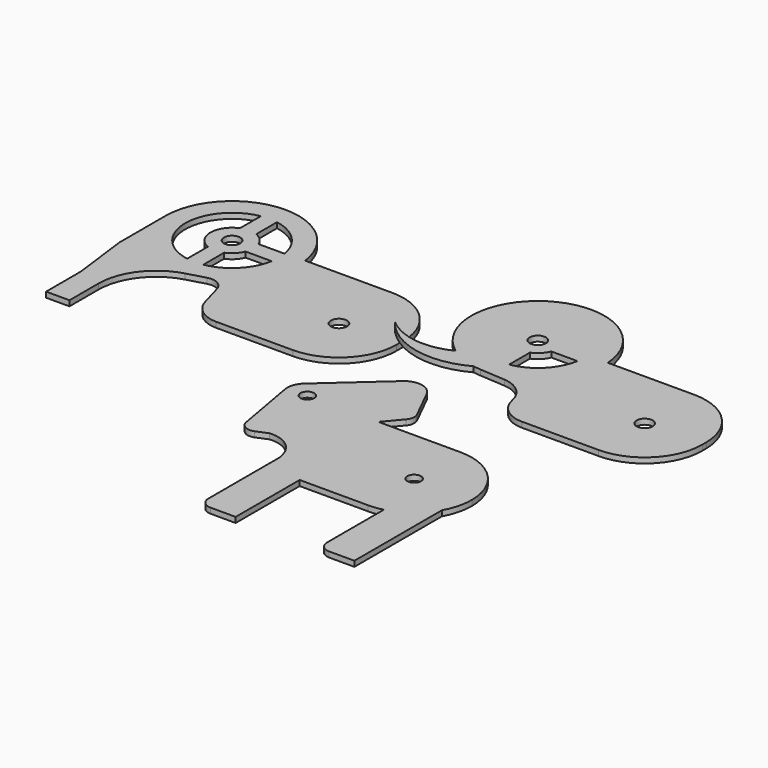
from build123d import *

# Parameters (mm, degrees)
F1_R     = 2.25
F2_DEPTH = 1.5
F3_R     = 2.25
F4_DEPTH = 1.5
F5_R     = 1.905
F6_DEPTH = 1.5


# Not quite as in the source:
# - a feature names something its author has since deleted; it is built from what else it names


with BuildPart() as f2:
    # F1 (on Top) → F2 (new body)
    with BuildSketch(Plane.XY):
        with BuildLine():
            Line((23.8478663564, 16.2219721824), (-0.3218308638, 16.2219721824))
            ThreePointArc((-0.3218308638, 16.2219721824), (-19.9050100488, 32.1794991216), (-37.1521336436, 13.7219721824))
            Line((-37.1521336436, 13.7219721824), (-37.1521336436, -2.2780278176))
            Line((-37.1521336436, -2.2780278176), (-35.1421336436, -18.2780278176))
            Line((-35.1421336436, -18.2780278176), (-35.1421336436, -30.2780278176))
            Line((-35.1421336436, -30.2780278176), (-28.6421336436, -30.2780278176))
            Line((-28.6421336436, -30.2780278176), (-28.6421336436, -20.1922246362))
            ThreePointArc((-28.6421336436, -20.1922246362), (-25.3982996099, -10.5340555633), (-16.9821049136, -4.7920736832))
            Line((-16.9821049136, -4.7920736832), (-11.9111882435, -3.3630206351))
            ThreePointArc((-11.9111882435, -3.3630206351), (-8.8710134123, -3.723464802), (-6.9761576878, -6.1280655559))
            Line((-6.9761576878, -6.1280655559), (-5.1951107108, -12.4480134526))
            ThreePointArc((-5.1951107108, -12.4480134526), (-2.3241197708, -16.6561108008), (2.5049647657, -18.2780278176))
            Line((2.5049647657, -18.2780278176), (23.8478663564, -18.2780278176))
            ThreePointArc((23.8478663564, -18.2780278176), (35.1615748554, -13.5917363166), (39.8478663564, -2.2780278176))
            Line((39.8478663564, -2.2780278176), (39.8478663564, 0.2219721824))
            ThreePointArc((39.8478663564, 0.2219721824), (35.1615748554, 11.5356806814), (23.8478663564, 16.2219721824))
        make_face()
        with Locations((23.8478663564, -2.2780278176)):
            Circle(F1_R, mode=Mode.SUBTRACT)
        with BuildLine():
            Line((-20.9021336436, 26.5257802097), (-20.9021336436, 19.2841210477))
            ThreePointArc((-20.9021336436, 19.2841210477), (-24.6521336436, 13.7219721824), (-20.9021336436, 8.1598233171))
            Line((-20.9021336436, 8.1598233171), (-20.9021336436, 0.9181641551))
            ThreePointArc((-20.9021336436, 0.9181641551), (-31.6521336436, 13.7219721824), (-20.9021336436, 26.5257802097))
        make_face(mode=Mode.SUBTRACT)
        with Locations((-18.6521336436, 13.7219721824)):
            Circle(F1_R, mode=Mode.SUBTRACT)
        with BuildLine():
            ThreePointArc((-16.4021336436, 8.1598233171), (-14.4094929565, 9.4793314953), (-13.0899847783, 11.4719721824))
            Line((-13.0899847783, 11.4719721824), (-5.8483256163, 11.4719721824))
            ThreePointArc((-5.8483256163, 11.4719721824), (-9.4597454882, 4.529584027), (-16.4021336436, 0.9181641551))
            Line((-16.4021336436, 0.9181641551), (-16.4021336436, 8.1598233171))
        make_face(mode=Mode.SUBTRACT)
        with BuildLine():
            ThreePointArc((-13.0899847783, 15.9719721824), (-14.4094929565, 17.9646128695), (-16.4021336436, 19.2841210477))
            Line((-16.4021336436, 19.2841210477), (-16.4021336436, 26.5257802097))
            ThreePointArc((-16.4021336436, 26.5257802097), (-9.4597454882, 22.9143603378), (-5.8483256163, 15.9719721824))
            Line((-5.8483256163, 15.9719721824), (-13.0899847783, 15.9719721824))
        make_face(mode=Mode.SUBTRACT)
    extrude(amount=F2_DEPTH)


with BuildPart() as f4:
    # F3 (on offset) → F4 (new body)
    with BuildSketch(Plane.XY.offset(3.5)):
        with BuildLine():
            Line((109.2000847661, 14.5111365989), (85.1578067274, 14.5111365989))
            ThreePointArc((85.1578067274, 14.5111365989), (85.1895122354, 13.8864939832), (85.2000847661, 13.2611365989))
            ThreePointArc((85.2000847661, 13.2611365989), (79.3391563377, -0.2482627146), (65.4699366786, -5.1979190563))
            Line((65.4699366786, -5.1979190563), (72.5876051284, -5.6722546017))
            ThreePointArc((72.5876051284, -5.6722546017), (77.0942321722, -7.4406386068), (79.7557246751, -11.4845633041))
            Line((79.7557246751, -11.4845633041), (80.1571076989, -12.9088490361))
            ThreePointArc((80.1571076989, -12.9088490361), (83.028098639, -17.1169463843), (87.8571831754, -18.7388634011))
            Line((87.8571831754, -18.7388634011), (109.2000847661, -18.7388634011))
            ThreePointArc((109.2000847661, -18.7388634011), (120.5137932651, -14.0525719001), (125.2000847661, -2.7388634011))
            Line((125.2000847661, -2.7388634011), (125.2000847661, -1.4888634011))
            ThreePointArc((125.2000847661, -1.4888634011), (120.5137932651, 9.8248450979), (109.2000847661, 14.5111365989))
        make_face()
        with Locations((109.2000847661, -2.7388634011)):
            Circle(F3_R, mode=Mode.SUBTRACT)
        with BuildLine():
            ThreePointArc((85.2000847661, 13.2611365989), (85.1895122354, 13.8864939832), (85.1578067274, 14.5111365989))
            ThreePointArc((85.1578067274, 14.5111365989), (57.7465852827, 29.4501713755), (55.8302690835, -1.7087367147))
            ThreePointArc((55.8302690835, -1.7087367147), (59.4538765607, -3.7606866479), (63.4446329394, -4.9501794822))
            ThreePointArc((63.4446329394, -4.9501794822), (64.4538667509, -5.1019923455), (65.4699366786, -5.1979190563))
            ThreePointArc((65.4699366786, -5.1979190563), (79.3391563377, -0.2482627146), (85.2000847661, 13.2611365989))
        make_face()
        with BuildLine():
            Line((68.9500847661, 0.4573285716), (68.9500847661, 7.6989877336))
            ThreePointArc((68.9500847661, 7.6989877336), (70.9427254533, 9.0184959118), (72.2622336315, 11.0111365989))
            Line((72.2622336315, 11.0111365989), (79.5038927935, 11.0111365989))
            ThreePointArc((79.5038927935, 11.0111365989), (75.8924729216, 4.0687484435), (68.9500847661, 0.4573285716))
        make_face(mode=Mode.SUBTRACT)
        with Locations((66.7000847661, 13.2611365989)):
            Circle(F3_R, mode=Mode.SUBTRACT)
        with BuildLine():
            ThreePointArc((63.4446329394, -4.9501794822), (59.4538765607, -3.7606866479), (55.8302690835, -1.7087367147))
            ThreePointArc((55.8302690835, -1.7087367147), (45.9967207055, -3.3960542374), (36.9400847661, 0.7900011357))
            ThreePointArc((36.9400847661, 0.7900011357), (49.1243667434, -7.0114058331), (63.4446329394, -4.9501794822))
        make_face()
    extrude(amount=F4_DEPTH)


with BuildPart() as f6:
    # F5 (on offset) → F6 (new body)
    with BuildSketch(Plane.XY.offset(3.5)):
        with BuildLine():
            Line((86.3721772379, -38.2815617886), (63.6372811817, -38.2815617886))
            Line((63.6372811817, -38.2815617886), (67.5948618811, -33.5741011418))
            ThreePointArc((67.5948618811, -33.5741011418), (68.2773760162, -31.9993262849), (67.9849045951, -30.3081131515))
            Line((67.9849045951, -30.3081131515), (63.6031002529, -21.4938680874))
            ThreePointArc((63.6031002529, -21.4938680874), (60.07017827, -18.8096304864), (55.7936149014, -19.9918635388))
            Line((55.7936149014, -19.9918635388), (39.7849043568, -34.3018614395))
            ThreePointArc((39.7849043568, -34.3018614395), (38.3906107486, -36.3986590518), (38.195076482, -38.9091134417))
            Line((38.195076482, -38.9091134417), (41.2990189026, -56.2805721912))
            ThreePointArc((41.2990189026, -56.2805721912), (42.8181559772, -58.3879184832), (45.412651037, -58.5193765789))
            Line((45.412651037, -58.5193765789), (48.4815553554, -57.232122972))
            ThreePointArc((48.4815553554, -57.232122972), (53.7537831872, -58.6006612256), (56.9278171468, -63.0272616916))
            Line((56.9278171468, -63.0272616916), (57.3292001707, -64.4515474235))
            ThreePointArc((57.3292001707, -64.4515474235), (60.2001911107, -68.6596447717), (65.0292756472, -70.2815617886))
            Line((65.0292756472, -70.2815617886), (67.3292001707, -70.2815617886))
            Line((67.3292001707, -70.2815617886), (86.3721772379, -70.2815617886))
            ThreePointArc((86.3721772379, -70.2815617886), (88.3662354627, -70.1568171187), (90.3292001707, -69.7845282631))
            ThreePointArc((90.3292001707, -69.7845282631), (96.117596449, -66.9711955264), (100.3292001707, -62.1047012385))
            ThreePointArc((100.3292001707, -62.1047012385), (101.8530100147, -58.324310425), (102.3721772379, -54.2815617886))
            ThreePointArc((102.3721772379, -54.2815617886), (97.6858857369, -42.9678532896), (86.3721772379, -38.2815617886))
        make_face()
        with Locations((43.8721772379, -38.2815617886)):
            Circle(F5_R, mode=Mode.SUBTRACT)
        with Locations((86.3721772379, -54.2815617886)):
            Circle(F5_R, mode=Mode.SUBTRACT)
        with BuildLine():
            Line((100.3292001707, -92.5101898611), (100.3292001707, -62.1047012385))
            ThreePointArc((100.3292001707, -62.1047012385), (96.117596449, -66.9711955264), (90.3292001707, -69.7845282631))
            Line((90.3292001707, -69.7845282631), (90.3292001707, -89.5101898611))
            ThreePointArc((90.3292001707, -89.5101898611), (91.2078798271, -91.6315102046), (93.3292001707, -92.5101898611))
            Line((93.3292001707, -92.5101898611), (100.3292001707, -92.5101898611))
        make_face()
        with BuildLine():
            Line((67.3292001707, -92.5101898611), (67.3292001707, -70.2815617886))
            Line((67.3292001707, -70.2815617886), (65.0292756472, -70.2815617886))
            ThreePointArc((65.0292756472, -70.2815617886), (60.2001911107, -68.6596447717), (57.3292001707, -64.4515474235))
            Line((57.3292001707, -64.4515474235), (57.3292001707, -89.5101898611))
            ThreePointArc((57.3292001707, -89.5101898611), (58.2078798271, -91.6315102046), (60.3292001707, -92.5101898611))
            Line((60.3292001707, -92.5101898611), (67.3292001707, -92.5101898611))
        make_face()
    extrude(amount=F6_DEPTH)


solid = Compound([f2.part, f4.part, f6.part])
